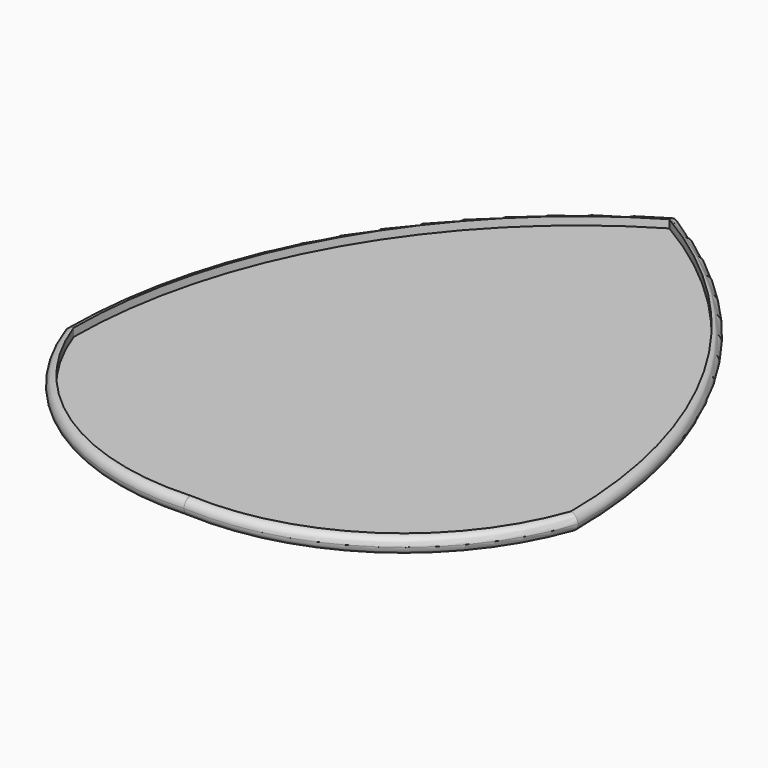
from build123d import *

# Parameters (mm, degrees)
F1_DEPTH = 0.8
F2_R     = 0.4
F3_R     = 0.39999
F4_W     = 4.168279469
F4_H     = 8
F5_DEPTH = 0.4
F6_DEPTH = 0.4


# Not quite as in the source:
# - a fillet or chamfer is up to 0.001 mm smaller than in the source, because OpenCascade refuses the exact size


with BuildPart() as f1:
    # F0 (on Top) → F1 (new body)
    with BuildSketch(Plane.XY):
        with BuildLine():
            ThreePointArc((0, 38.1792416396), (-9.2970452561, 28.8821963835), (-12.7, 16.1821963835))
            ThreePointArc((-12.7, 16.1821963835), (-7.7676026835, 9.8183978835), (0, 7.6992416396))
            ThreePointArc((0, 7.6992416396), (7.7676026835, 9.8183978835), (12.7, 16.1821963835))
            ThreePointArc((12.7, 16.1821963835), (9.3014350381, 28.8847308253), (0, 38.1792416396))
        make_face()
    extrude(amount=F1_DEPTH)

    # F2
    f2_edges = [f1.edges().sort_by_distance(p)[0] for p in [
        (-9.297045, 28.882196, 0.8),
        (-7.767603, 9.818398, 0.8),
        (7.767603, 9.818398, 0.8),
        (9.301435, 28.884731, 0.8),
    ]]
    fillet(f2_edges, radius=F2_R)

    # F3 (radius 0.4 in the source; OpenCascade refuses exactly that, so slightly less here)
    f3_edges = [f1.edges().sort_by_distance(p)[0] for p in [
        (7.767603, 9.818398, 0),
        (9.301435, 28.884731, 0),
        (-7.767603, 9.818398, 0),
        (-9.297045, 28.882196, 0),
    ]]
    fillet(f3_edges, radius=F3_R)

    # F4 (on Top) + F1_face (on face) + F1_face1 (on face) → F5 (cut)
    with BuildSketch(Plane.XY):
        Polygon((1.9827442754, 19.357689971), (-4.0172557246, 19.357689971), (-1.0172557246, 14.1615375483), align=None)
        with BuildLine():
            Line((-9.0172557246, 19.357689971), (-9.0172557246, 15.857689971))
            ThreePointArc((-9.0172557246, 15.857689971), (-6.5423819904, 16.8828162368), (-5.5172557246, 19.357689971))
            Line((-5.5172557246, 19.357689971), (-9.0172557246, 19.357689971))
        make_face()
        Polygon((-1.0172557246, 25.5538423937), (-4.0172557246, 20.357689971), (1.9827442754, 20.357689971), align=None)
        with Locations((5.56688401, 15.357689971)):
            Rectangle(F4_W, F4_H)
        with BuildLine():
            Line((-9.0172557246, 20.357689971), (-5.5172557246, 20.357689971))
            ThreePointArc((-5.5172557246, 20.357689971), (-6.5423819904, 22.8325637051), (-9.0172557246, 23.857689971))
            Line((-9.0172557246, 23.857689971), (-9.0172557246, 20.357689971))
        make_face()
        with Locations((5.56688401, 24.357689971)):
            Rectangle(F4_W, F4_H)
    with BuildSketch(Plane(origin=(0.0014081173, 21.2624606857, 0.8), x_dir=(1, 0, 0), z_dir=(0, 0, 1))):
        with BuildLine():
            ThreePointArc((-0.0012370935, 16.4537632815), (-8.9926932828, 7.3490618207), (-12.3013148115, -5.0119614651))
            ThreePointArc((-12.3013148115, -5.0119614651), (-7.5186387645, -11.1302175722), (-0.0238816927, -13.1638508721))
            add(Edge.make_bspline(
                [(-0.0238816927, -13.1638508721), (-0.0125655835, -13.1632140826), (-0.0014081173, -13.1622533084), (0.009749349, -13.1632140826), (0.0210654582, -13.1638508721)],
                knots=[0, 0, 0, 0, 0, 1, 1, 1, 1, 1], degree=4))
            ThreePointArc((0.0210654582, -13.1638508721), (7.5158860187, -11.1301754171), (12.2985497378, -5.0118178891))
            ThreePointArc((12.2985497378, -5.0118178891), (8.9943044567, 7.3515302466), (-0.0012370935, 16.4537632815))
        make_face()
    with BuildSketch(Plane(origin=(0.001408117, 21.262461098, 0), x_dir=(1, 0, 0), z_dir=(0, 0, -1))):
        with BuildLine():
            ThreePointArc((12.2985597415, 5.0118200202), (7.5158922747, 11.1301836793), (0.0210648966, 13.1638612686))
            add(Edge.make_bspline(
                [(0.0210648966, 13.1638612686), (0.0097490703, 13.1632244951), (-0.001408117, 13.1622637449), (-0.0125653043, 13.1632244951), (-0.0238811306, 13.1638612686)],
                knots=[0, 0, 0, 0, 0, 1, 1, 1, 1, 1], degree=4))
            ThreePointArc((-0.0238811306, 13.1638612686), (-7.5186450215, 11.1302258334), (-12.301324816, 5.0119635927))
            ThreePointArc((-12.301324816, 5.0119635927), (-8.9927009274, -7.3490681805), (-0.0012370975, -16.4537744762))
            ThreePointArc((-0.0012370975, -16.4537744762), (8.9943121009, -7.3515366081), (12.2985597415, 5.0118200202))
        make_face()
    extrude(amount=-F5_DEPTH, dir=(0, 0, 1), mode=Mode.SUBTRACT)

    # F4 (on Top) → F6 (join)
    with BuildSketch(Plane.XY):
        with BuildLine():
            Line((-9.0172557246, 19.357689971), (-9.0172557246, 15.857689971))
            ThreePointArc((-9.0172557246, 15.857689971), (-6.5423819904, 16.8828162368), (-5.5172557246, 19.357689971))
            Line((-5.5172557246, 19.357689971), (-9.0172557246, 19.357689971))
        make_face()
        with BuildLine():
            Line((-9.0172557246, 20.357689971), (-5.5172557246, 20.357689971))
            ThreePointArc((-5.5172557246, 20.357689971), (-6.5423819904, 22.8325637051), (-9.0172557246, 23.857689971))
            Line((-9.0172557246, 23.857689971), (-9.0172557246, 20.357689971))
        make_face()
        Polygon((-1.0172557246, 25.5538423937), (-4.0172557246, 20.357689971), (1.9827442754, 20.357689971), align=None)
        Polygon((1.9827442754, 19.357689971), (-4.0172557246, 19.357689971), (-1.0172557246, 14.1615375483), align=None)
        with Locations((5.56688401, 24.357689971)):
            Rectangle(F4_W, F4_H)
        with Locations((5.56688401, 15.357689971)):
            Rectangle(F4_W, F4_H)
    extrude(amount=-F6_DEPTH)


solid = f1.part
